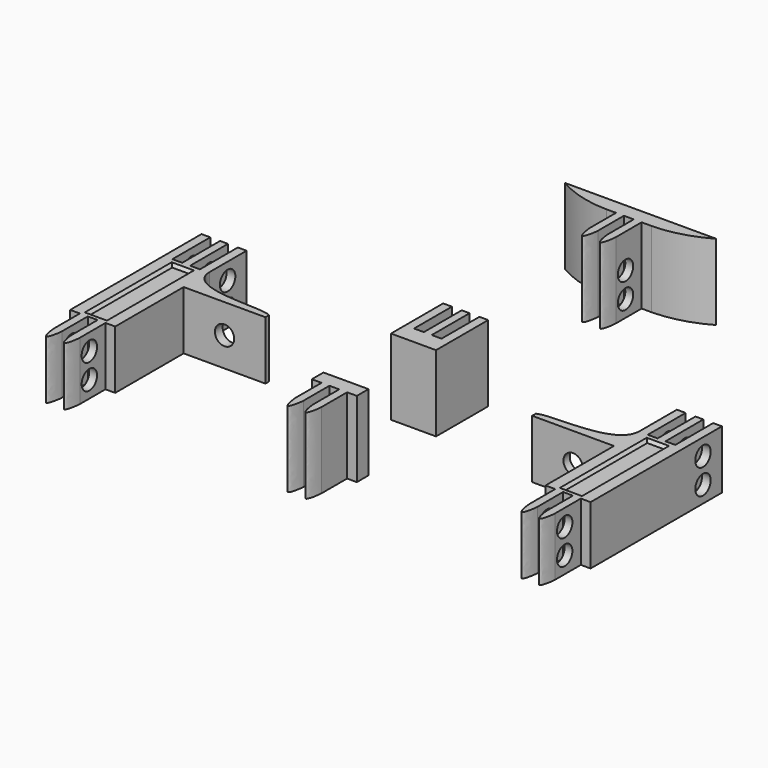
from build123d import *

# Parameters (mm, degrees)
F1_DEPTH  = 10
F2_DEPTH  = 13
F4_D      = 3.3
F8_D      = 3.3
F8_2_D    = 3.3
F9_W      = 1.9
F9_H      = 1.9
F10_DEPTH = 0.5
F10_TAPER = 40
F13_DEPTH = 13


# Not quite as in the source:
# - a feature names something its author has since deleted; it is built from what else it names


with BuildPart() as f1:
    # F0 (on Top) → F1 (new body)
    with BuildSketch(Plane.XY):
        with BuildLine():
            add(Edge.make_bspline(
                [(-5.836743505, 0), (-4.2651791979, 0.5970813636), (-3.18, 1.5815938376), (-3.18, 3.2431164291)],
                knots=[10.3584422761, 10.3584422761, 10.3584422761, 10.3584422761, 14.7923904362, 14.7923904362, 14.7923904362, 14.7923904362], degree=3))
            Line((-5.836743505, 0), (-3.18, 0))
            Line((-3.18, 0), (-3.18, 3.2431164291))
        make_face()
        with BuildLine():
            Line((-3.18, 0), (-5.836743505, 0))
            add(Edge.make_bspline(
                [(-17.18, -1.5333691845), (-15.8341479718, -0.675290137), (-9.5081797893, -1.3948816304), (-5.836743505, 0)],
                knots=[0, 0, 0, 0, 10.3584422761, 10.3584422761, 10.3584422761, 10.3584422761], degree=3))
            Line((-17.18, -1.5333691845), (-17.18, -2.3))
            Line((-17.18, -2.3), (-3.18, -2.3))
            Line((-3.18, -2.3), (-3.18, -14.440753624))
            Line((-3.18, -14.440753624), (4.53, -14.440753624))
            Line((4.53, -14.440753624), (4.53, 0))
            Line((4.53, 0), (-3.18, 0))
        make_face()
        with BuildLine():
            Line((4.53, -16.940753624), (4.53, -14.440753624))
            Line((4.53, -14.440753624), (-3.18, -14.440753624))
            Line((-3.18, -14.440753624), (-3.18, -16.940753624))
            Line((-3.18, -16.940753624), (-1.515, -16.940753624))
            Line((-1.515, -16.940753624), (-1.515, -22.440753624))
            add(Edge.make_bspline(
                [(-1.515, -22.440753624), (-1.515, -23.0624348587), (-1.1775, -24.940753624), (-0.84, -24.940753624)],
                knots=[0, 0, 0, 0, 0.5, 0.5, 0.5, 0.5], degree=3))
            add(Edge.make_bspline(
                [(-0.84, -24.940753624), (-0.5025, -24.940753624), (-0.165, -23.0624348587), (-0.165, -22.440753624)],
                knots=[0.5, 0.5, 0.5, 0.5, 1, 1, 1, 1], degree=3))
            Line((-0.165, -22.440753624), (-0.165, -16.940753624))
            Line((-0.165, -16.940753624), (1.515, -16.940753624))
            Line((1.515, -16.940753624), (1.515, -22.440753624))
            add(Edge.make_bspline(
                [(2.19, -24.940753624), (1.8525, -24.940753624), (1.515, -23.0624348587), (1.515, -22.440753624)],
                knots=[0.5, 0.5, 0.5, 0.5, 1, 1, 1, 1], degree=3))
            add(Edge.make_bspline(
                [(2.865, -22.440753624), (2.865, -23.0624348587), (2.5275, -24.940753624), (2.19, -24.940753624)],
                knots=[0, 0, 0, 0, 0.5, 0.5, 0.5, 0.5], degree=3))
            Line((2.865, -22.440753624), (2.865, -16.940753624))
            Line((2.865, -16.940753624), (4.53, -16.940753624))
        make_face()
        Polygon((-3.18, 3.2431164291), (-3.18, 0), (4.53, 0), (4.53, 11.159246376), (3.03, 11.159246376), (3.03, 3.059246376), (1.35, 3.059246376), (1.35, 11.159246376), (0, 11.159246376), (0, 3.059246376), (-1.68, 3.059246376), (-1.68, 11.159246376), (-3.18, 11.159246376), align=None)
    extrude(amount=F1_DEPTH)

    # F4 (through all)
    with Locations(Plane.XZ.offset(2.3)):
        with Locations((-10.18, 5)):
            Hole(F4_D / 2)

    # F8 (through all)
    with Locations(Plane(origin=(-3.18, 0, 0), x_dir=(0, -1, 0), z_dir=(-1, 0, 0))):
        with Locations((-7.109246376, 7.15), (-7.109246376, 2.85), (20.3907460467, 7.15), (20.3907460467, 2.85)):
            Hole(F8_D / 2)

    # F9 (on face) → F10 (cut)
    with BuildSketch(Plane.XY.offset(10)):
        with Locations((-0.3, -15.3403911533)):
            Rectangle(F9_W, F9_H)
        with Locations((1.6, -13.4403911533)):
            Rectangle(F9_W, F9_H)
        with Locations((-0.3, -11.5403911533)):
            Rectangle(F9_W, F9_H)
        with Locations((1.6, -9.6403911533)):
            Rectangle(F9_W, F9_H)
        with Locations((-0.3, -7.7403911533)):
            Rectangle(F9_W, F9_H)
        with Locations((1.6, -5.8403911533)):
            Rectangle(F9_W, F9_H)
        with Locations((-0.3, -3.9403911533)):
            Rectangle(F9_W, F9_H)
        with Locations((1.6, -2.0403911533)):
            Rectangle(F9_W, F9_H)
        with Locations((1.6, -15.3403911533)):
            Rectangle(F9_W, F9_H)
        with Locations((-0.3, -13.4403911533)):
            Rectangle(F9_W, F9_H)
        with Locations((1.6, -11.5403911533)):
            Rectangle(F9_W, F9_H)
        with Locations((-0.3, -9.6403911533)):
            Rectangle(F9_W, F9_H)
        with Locations((1.6, -7.7403911533)):
            Rectangle(F9_W, F9_H)
        with Locations((-0.3, -5.8403911533)):
            Rectangle(F9_W, F9_H)
        with Locations((1.6, -3.9403911533)):
            Rectangle(F9_W, F9_H)
        Polygon((-1.25, -1.0903911533), (-1.25, -1.3), (-1.25, -2.9903911533), (0.65, -2.9903911533), (0.65, -1.0903911533), align=None)
        Polygon((-1.25, 2.309246376), (-1.25, -1.0903911533), (0.65, -1.0903911533), (2.55, -1.0903911533), (2.55, 2.309246376), align=None)
    extrude(amount=-F10_DEPTH, taper=F10_TAPER, mode=Mode.SUBTRACT)


with BuildPart() as f2:
    # F0 (on Top) → F2 (new body)
    with BuildSketch(Plane.XY):
        with BuildLine():
            Line((-3.18, -16.940753624), (-3.18, -14.440753624))
            Line((-3.18, -14.440753624), (-12.2665563866, -14.440753624))
            ThreePointArc((-12.2665563866, -14.440753624), (-7.8858323009, -16.2815764499), (-3.18, -16.940753624))
        make_face()
        with BuildLine():
            Line((4.53, -16.940753624), (4.53, -14.440753624))
            Line((4.53, -14.440753624), (-3.18, -14.440753624))
            Line((-3.18, -14.440753624), (-3.18, -16.940753624))
            Line((-3.18, -16.940753624), (-1.515, -16.940753624))
            Line((-1.515, -16.940753624), (-1.515, -22.440753624))
            add(Edge.make_bspline(
                [(-1.515, -22.440753624), (-1.515, -23.0624348587), (-1.1775, -24.940753624), (-0.84, -24.940753624)],
                knots=[0, 0, 0, 0, 0.5, 0.5, 0.5, 0.5], degree=3))
            add(Edge.make_bspline(
                [(-0.84, -24.940753624), (-0.5025, -24.940753624), (-0.165, -23.0624348587), (-0.165, -22.440753624)],
                knots=[0.5, 0.5, 0.5, 0.5, 1, 1, 1, 1], degree=3))
            Line((-0.165, -22.440753624), (-0.165, -16.940753624))
            Line((-0.165, -16.940753624), (1.515, -16.940753624))
            Line((1.515, -16.940753624), (1.515, -22.440753624))
            add(Edge.make_bspline(
                [(2.19, -24.940753624), (1.8525, -24.940753624), (1.515, -23.0624348587), (1.515, -22.440753624)],
                knots=[0.5, 0.5, 0.5, 0.5, 1, 1, 1, 1], degree=3))
            add(Edge.make_bspline(
                [(2.865, -22.440753624), (2.865, -23.0624348587), (2.5275, -24.940753624), (2.19, -24.940753624)],
                knots=[0, 0, 0, 0, 0.5, 0.5, 0.5, 0.5], degree=3))
            Line((2.865, -22.440753624), (2.865, -16.940753624))
            Line((2.865, -16.940753624), (4.53, -16.940753624))
        make_face()
        with BuildLine():
            Line((13.6165563866, -14.440753624), (4.53, -14.440753624))
            Line((4.53, -14.440753624), (4.53, -16.940753624))
            ThreePointArc((4.53, -16.940753624), (9.2358323009, -16.2815764499), (13.6165563866, -14.440753624))
        make_face()
    extrude(amount=F2_DEPTH)

    # F8#2 (through all)
    with Locations(Plane(origin=(-3.18, 0, 0), x_dir=(0, -1, 0), z_dir=(-1, 0, 0))):
        with Locations((-7.109246376, 7.15), (-7.109246376, 2.85), (20.3907460467, 7.15), (20.3907460467, 2.85)):
            Hole(F8_2_D / 2)


with BuildPart() as f1_1:
    # F11: moved
    add(f1.part.moved(Location((40, 0, 0))))


with BuildPart() as f12_1:
    # F12: instance of F1
    add(f1_1.part.mirror(Plane.YZ))


with BuildPart() as f13:
    # F0 (on Top) → F13 (new body)
    with BuildSketch(Plane.XY):
        with BuildLine():
            Line((4.53, -16.940753624), (4.53, -14.440753624))
            Line((4.53, -14.440753624), (-3.18, -14.440753624))
            Line((-3.18, -14.440753624), (-3.18, -16.940753624))
            Line((-3.18, -16.940753624), (-1.515, -16.940753624))
            Line((-1.515, -16.940753624), (-1.515, -22.440753624))
            add(Edge.make_bspline(
                [(-1.515, -22.440753624), (-1.515, -23.0624348587), (-1.1775, -24.940753624), (-0.84, -24.940753624)],
                knots=[0, 0, 0, 0, 0.5, 0.5, 0.5, 0.5], degree=3))
            add(Edge.make_bspline(
                [(-0.84, -24.940753624), (-0.5025, -24.940753624), (-0.165, -23.0624348587), (-0.165, -22.440753624)],
                knots=[0.5, 0.5, 0.5, 0.5, 1, 1, 1, 1], degree=3))
            Line((-0.165, -22.440753624), (-0.165, -16.940753624))
            Line((-0.165, -16.940753624), (1.515, -16.940753624))
            Line((1.515, -16.940753624), (1.515, -22.440753624))
            add(Edge.make_bspline(
                [(2.19, -24.940753624), (1.8525, -24.940753624), (1.515, -23.0624348587), (1.515, -22.440753624)],
                knots=[0.5, 0.5, 0.5, 0.5, 1, 1, 1, 1], degree=3))
            add(Edge.make_bspline(
                [(2.865, -22.440753624), (2.865, -23.0624348587), (2.5275, -24.940753624), (2.19, -24.940753624)],
                knots=[0, 0, 0, 0, 0.5, 0.5, 0.5, 0.5], degree=3))
            Line((2.865, -22.440753624), (2.865, -16.940753624))
            Line((2.865, -16.940753624), (4.53, -16.940753624))
        make_face()
    extrude(amount=F13_DEPTH)


with BuildPart() as f13b:
    # F0 (on Top) → F13, piece 2 (new body)
    with BuildSketch(Plane.XY):
        Polygon((-3.18, 3.2431164291), (-3.18, 0), (4.53, 0), (4.53, 11.159246376), (3.03, 11.159246376), (3.03, 3.059246376), (1.35, 3.059246376), (1.35, 11.159246376), (0, 11.159246376), (0, 3.059246376), (-1.68, 3.059246376), (-1.68, 11.159246376), (-3.18, 11.159246376), align=None)
    extrude(amount=F13_DEPTH)


with BuildPart() as f2_1:
    # F14: moved
    add(f2.part.moved(Location((0, 63, 0))))


solid = Compound([f1_1.part, f12_1.part, f13.part, f13b.part, f2_1.part])
